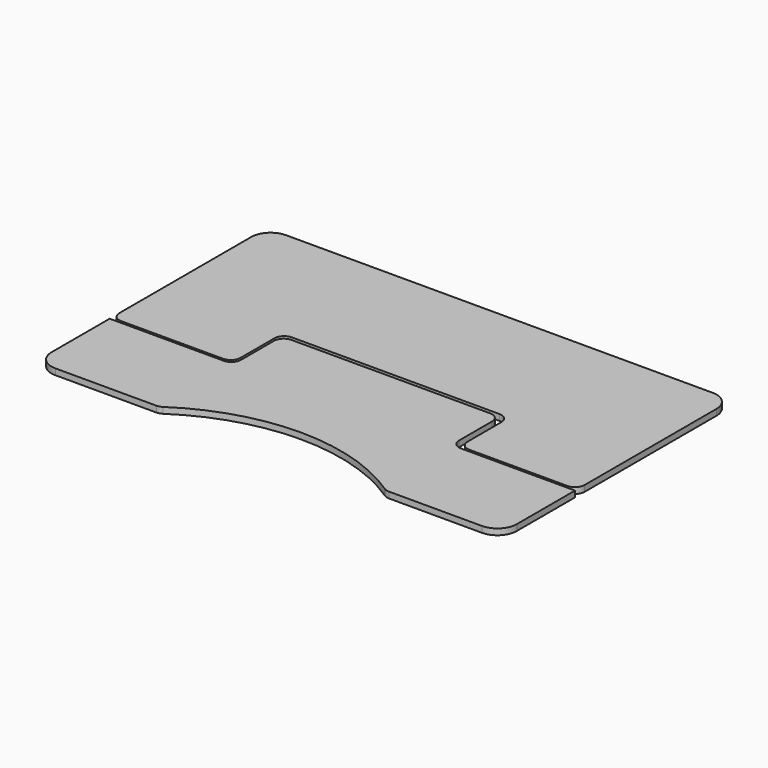
from build123d import *

# Parameters (mm, degrees)
F1_DEPTH = 15.875
F2_DEPTH = 15.875


# Not quite as in the source:
# - a length typed as a fraction of an inch, garbled in the dataset ("3 / 203.2 mm" for 3/8 in), is restored


with BuildPart() as f1:
    # F0 (on Top) → F1 (new body)
    with BuildSketch(Plane.XY):
        with BuildLine():
            Line((-558.8, -377.825), (-294.0262573309, -377.825))
            ThreePointArc((-294.0262573309, -377.825), (-286.6751320609, -376.7379791935), (-279.9532056979, -373.569957265))
            ThreePointArc((-279.9532056979, -373.569957265), (10.5547887247, -285.7337179487), (301.0627831473, -373.569957265))
            ThreePointArc((301.0627831473, -373.569957265), (307.7847095103, -376.7379791935), (315.1358347803, -377.825))
            Line((315.1358347803, -377.825), (558.8, -377.825))
            ThreePointArc((558.8, -377.825), (594.7210244843, -362.9460244843), (609.6, -327.025))
            Line((609.6, -327.025), (609.6, -136.5972012281))
            Line((609.6, -136.5972012281), (609.6, -136.525))
            Line((609.6, -136.525), (311.1499893665, -136.525))
            ThreePointArc((311.1499893665, -136.525), (293.1894771244, -129.0855122421), (285.7499893665, -111.125))
            Line((285.7499893665, -111.125), (285.7499893665, -3.1749994576))
            ThreePointArc((285.7499893665, -3.1749994576), (278.3105016087, 14.7855127845), (260.3499893665, 22.2250005424))
            Line((260.3499893665, 22.2250005424), (-260.35, 22.2250005424))
            ThreePointArc((-260.35, 22.2250005424), (-278.3105122421, 14.7855127845), (-285.75, -3.1749994576))
            Line((-285.75, -3.1749994576), (-285.75, -111.125))
            ThreePointArc((-285.75, -111.125), (-293.1894877579, -129.0855122421), (-311.15, -136.525))
            Line((-311.15, -136.525), (-609.6, -136.525))
            Line((-609.6, -136.525), (-609.6, -327.025))
            ThreePointArc((-609.6, -327.025), (-594.7210244843, -362.9460244843), (-558.8, -377.825))
        make_face()
    extrude(amount=F1_DEPTH)


with BuildPart() as f2:
    # F0 (on Top) → F2 (new body)
    with BuildSketch(Plane.XY):
        with BuildLine():
            ThreePointArc((609.6, 327.025), (594.7210244843, 362.9460244843), (558.8, 377.825))
            Line((558.8, 377.825), (-558.8, 377.825))
            ThreePointArc((-558.8, 377.825), (-594.7210244843, 362.9460244843), (-609.6, 327.025))
            Line((-609.6, 327.025), (-609.6, -104.775))
            ThreePointArc((-609.6, -104.775), (-602.1605122421, -122.7355122421), (-584.2, -130.175))
            Line((-584.2, -130.175), (-317.5, -130.175))
            ThreePointArc((-317.5, -130.175), (-299.5394877579, -122.7355122421), (-292.1, -104.775))
            Line((-292.1, -104.775), (-292.1, 6.3662820513))
            ThreePointArc((-292.1, 6.3662820513), (-284.6605122421, 24.3267942934), (-266.7, 31.7662820513))
            Line((-266.7, 31.7662820513), (277.2547887247, 31.7662820513))
            ThreePointArc((277.2547887247, 31.7662820513), (295.2153009668, 24.3267942934), (302.6547887247, 6.3662820513))
            Line((302.6547887247, 6.3662820513), (302.6547887247, -104.775))
            ThreePointArc((302.6547887247, -104.775), (310.0942764826, -122.7355122421), (328.0547887247, -130.175))
            Line((328.0547887247, -130.175), (584.2, -130.175))
            ThreePointArc((584.2, -130.175), (602.1605122421, -122.7355122421), (609.6, -104.775))
            Line((609.6, -104.775), (609.6, 327.025))
        make_face()
    extrude(amount=F2_DEPTH)


solid = Compound([f1.part, f2.part])
